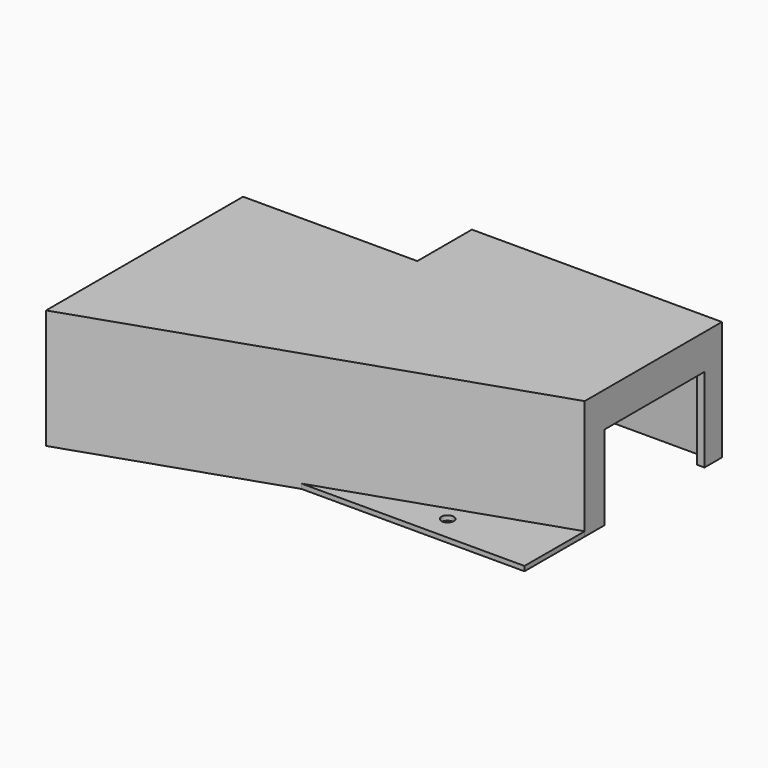
from build123d import *

# Parameters (mm, degrees)
F1_DEPTH    = 63
F2_DEPTH    = 2.5
F3_T        = 4
F3_T3_DEPTH = 132.2533825366
F3_T5_DEPTH = 10.5
F3_T7_DEPTH = 71
F4_W        = 44
F4_H        = 52
F4_W_2      = 45
F5_DEPTH    = 4.5
F7_DEPTH    = 5
F9_DEPTH    = 25


# Not quite as in the source:
# - a shell that OpenCascade refuses in one call is made with other operations: the cavity is built on its own and cut out


with BuildPart() as f1:
    # F0 (on Top) → F1 (new body)
    with BuildSketch(Plane.XY):
        Polygon((26.2132732272, -24.0364130735), (26.2132732272, 29.9635869265), (-65.7867267728, 29.9635869265), (-65.7867267728, -100.0364130735), (26.2132732272, -69.0364130735), align=None)
        Polygon((158.2132732272, 65.9635869265), (26.2132732272, 65.9635869265), (26.2132732272, 29.9635869265), (26.2132732272, -24.0364130735), (26.2132732272, -69.0364130735), (40.4647773284, -64.234275822), (158.2132732272, -24.558152204), align=None)
    extrude(amount=F1_DEPTH)

    # F0 (on Top) → F2 (join)
    with BuildSketch(Plane.XY):
        Polygon((158.2132732272, 65.9635869265), (26.2132732272, 65.9635869265), (26.2132732272, 29.9635869265), (26.2132732272, -24.0364130735), (26.2132732272, -69.0364130735), (40.4647773284, -64.234275822), (158.2132732272, -24.558152204), align=None)
        Polygon((26.2132732272, -24.0364130735), (26.2132732272, 29.9635869265), (-65.7867267728, 29.9635869265), (-65.7867267728, -100.0364130735), (26.2132732272, -69.0364130735), align=None)
        Polygon((158.1303410754, -64.234275822), (158.2132732272, -24.558152204), (40.4647773284, -64.234275822), align=None)
    extrude(amount=F2_DEPTH)

    # F3: shell of thickness 4, made by hand


with BuildPart() as f3_core1:
    # F3_t2: copy of F1
    add(f1.part)

    # the walls: a layer under each face that stays
    f3_faces = [f3_core1.faces().sort_by_distance(p)[0] for p in [
        (46.2132732272, -62.2972826388, 31.5),
        (99.2975592019, -64.234275822, 1.25),
        (158.1718071513, -44.396214013, 1.25),
        (99.3390252778, -57.6215885524, 2.5),
        (158.2132732272, 20.7027173612, 31.5),
        (92.2132732272, 65.9635869265, 31.5),
        (26.2132732272, 47.9635869265, 31.5),
        (-19.7867267728, 29.9635869265, 31.5),
        (46.2132732272, -17.0364130735, 63),
        (-65.7867267728, -35.0364130735, 31.5),
    ]]
    thicken(f3_faces, amount=-F3_T, mode=Mode.SUBTRACT)

    # F3_s4 → F3_t3 (cut)
    with BuildSketch(Plane(origin=(13.1110220732, 4.4178443942, 0), x_dir=(0, 0, 1), z_dir=(0.9476482128, 0.3193162456, 0))):
        Polygon((2.54, 73.8325574618), (2.5, 69.7925574618), (-1.5, 69.7925574618), (-1.5, 73.7925574618), align=None)
    extrude(amount=F3_T3_DEPTH, mode=Mode.SUBTRACT)

    # F3_s6 → F3_t5 (cut)
    with BuildSketch(Plane.XY.offset(-4)):
        Polygon((40.4775499783, -64.3121817506), (39.1875123459, -60.4436829707), (39.8089787227, -60.234275822), (40.4647773284, -60.234275822), align=None)
    extrude(amount=F3_T5_DEPTH, mode=Mode.SUBTRACT)

    # F3_s8 → F3_t7 (cut)
    with BuildSketch(Plane.XY.offset(-4)):
        Polygon((26.1732732272, 30.0035869265), (30.2132732272, 29.9635869265), (30.2132732272, 25.9635869265), (26.2132732272, 25.9635869265), align=None)
    extrude(amount=F3_T7_DEPTH, mode=Mode.SUBTRACT)


with BuildPart() as f1_1:
    add(f1.part)

    # what is left inside the walls is the cavity
    f3_cavity = [f3_core1.part.solids().sort_by_distance(p)[0] for p in [
        (46.213273, -42.323879, 0.04),
    ]]
    add(f3_cavity, mode=Mode.SUBTRACT)

    # F4 (on face) → F5 (cut)
    with BuildSketch(Plane(origin=(-65.7867267728, 0, 0), x_dir=(0, -1, 0), z_dir=(-1, 0, 0))):
        with Locations((68.8298759162, 26)):
            Rectangle(F4_W, F4_H)
        with Locations((3.3298759162, 26)):
            Rectangle(F4_W_2, F4_H)
    extrude(amount=-F5_DEPTH, mode=Mode.SUBTRACT)

    # F6 (on face) → F7 (cut)
    with BuildSketch(Plane.YZ.offset(158.2132732272)):
        Polygon((36.0559523106, 44.5), (-11.5364130735, 44.5), (-11.5364130735, 0), (54.4635869265, 0), (54.4635869265, 44.5), align=None)
    extrude(amount=-F7_DEPTH, mode=Mode.SUBTRACT)

    # F8 (on face) → F9 (cut)
    with BuildSketch(Plane.XY.offset(2.5)):
        with BuildLine():
            ThreePointArc((107.1575140418, -54.484275822), (109.4556110807, -53.5323728609), (110.4075140418, -51.234275822))
            Line((110.4075140418, -51.234275822), (107.1575140418, -51.234275822))
            Line((107.1575140418, -51.234275822), (107.1575140418, -54.484275822))
        make_face()
        with BuildLine():
            Line((107.1575140418, -51.234275822), (110.4075140418, -51.234275822))
            ThreePointArc((110.4075140418, -51.234275822), (104.859417003, -48.9361787832), (107.1575140418, -54.484275822))
            Line((107.1575140418, -54.484275822), (107.1575140418, -51.234275822))
        make_face()
    extrude(amount=-F9_DEPTH, mode=Mode.SUBTRACT)


solid = f1_1.part
